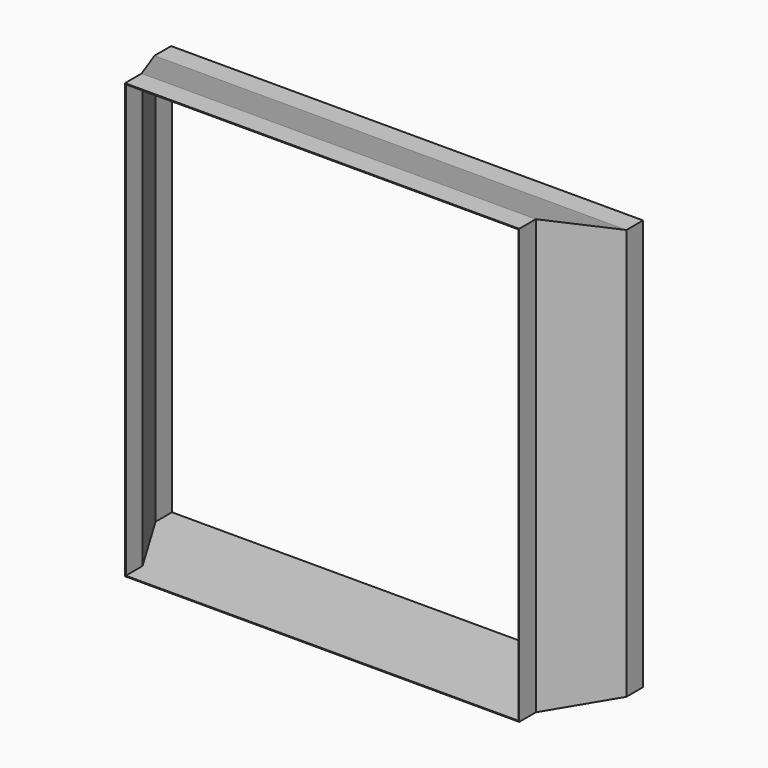
from build123d import *

# Parameters (mm, degrees)
F0_W        = 1462
F0_H        = 1610
F1_DEPTH    = 77
F3_W        = 1750
F3_H        = 1524
F4_DEPTH    = 77
F1_FACE_W   = 1462
F1_FACE_H   = 1610
F4_FACE_W   = 1750
F4_FACE_H   = 1524
F6_T        = 3
F6_T3_DEPTH = 1756
F6_T5_DEPTH = 1616


# Not quite as in the source:
# - a shell that OpenCascade refuses in one call is made with other operations: the cavity is built on its own and cut out


with BuildPart() as f1:
    # F0 (on Front) → F1 (new body)
    with BuildSketch(Plane.XZ):
        with Locations((0, 805)):
            Rectangle(F0_W, F0_H)
    extrude(amount=-F1_DEPTH)



with BuildPart() as f4:
    # F3 (on offset) → F4 (new body)
    with BuildSketch(Plane(origin=(0, 317, 0), x_dir=(-1, 0, 0), z_dir=(0, 1, 0))):
        with Locations((0, 762)):
            Rectangle(F3_W, F3_H)
    extrude(amount=F4_DEPTH)


with BuildPart() as f1_1:
    add(f1.part)

    add(f4.part)  # F5 merges F4
    # F1_face (on face) → F5 section 0
    with BuildSketch(Plane(origin=(0, 77, 805), x_dir=(1, 0, 0), z_dir=(0, 1, 0))):
        Rectangle(F1_FACE_W, F1_FACE_H)
    # F4_face (on face) → F5 section 1
    with BuildSketch(Plane(origin=(0, 317, 762), x_dir=(-1, 0, 0), z_dir=(0, -1, 0))):
        Rectangle(F4_FACE_W, F4_FACE_H)
    loft()

    # F6: shell of thickness 3, made by hand


with BuildPart() as f6_core1:
    # F6_t2: copy of F1
    add(f1_1.part)

    # the walls: a layer under each face that stays
    f6_faces = [f6_core1.faces().sort_by_distance(p)[0] for p in [
        (0, 197, 0),
        (875, 355.5, 762),
        (-875, 355.5, 762),
        (0, 355.5, 1524),
        (803, 197, 783.5),
        (-803, 197, 783.5),
        (-731, 38.5, 805),
        (731, 38.5, 805),
        (0, 197, 1567),
        (0, 38.5, 1610),
    ]]
    thicken(f6_faces, amount=-F6_T, mode=Mode.SUBTRACT)

    # F6_s4 → F6_t3 (cut)
    with BuildSketch(Plane.YZ.offset(-878)):
        Polygon((317.010119904, 1524.0582415924), (317, 1521), (316.4787279914, 1521), (315.988009604, 1521.1758407555), align=None)
    extrude(amount=F6_T3_DEPTH, mode=Mode.SUBTRACT)

    # F6_s6 → F6_t5 (cut)
    with BuildSketch(Plane.XY.offset(-3)):
        Polygon((731.0557247878, 76.9845651273), (728.4275212229, 78.5434872663), (728, 77.8309518948), (728, 77), align=None)
        Polygon((-731.0557247878, 76.9845651273), (-728.4275212229, 78.5434872663), (-728, 77.8309518948), (-728, 77), align=None)
    extrude(amount=F6_T5_DEPTH, mode=Mode.SUBTRACT)


with BuildPart() as f1_2:
    add(f1_1.part)

    # what is left inside the walls is the cavity
    f6_cavity = [f6_core1.part.solids().sort_by_distance(p)[0] for p in [
        (0, 393.97, 509),
    ]]
    add(f6_cavity, mode=Mode.SUBTRACT)


solid = f1_2.part
